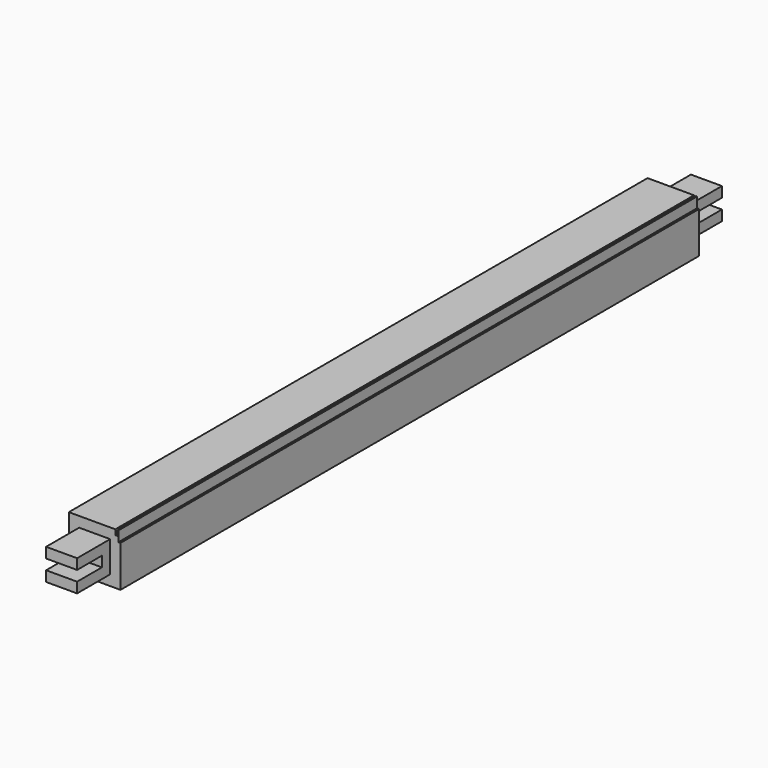
from build123d import *

# Parameters (mm, degrees)
F0_W      = 50
F0_H      = 50
F1_DEPTH  = 700
F3_W      = 30
F3_H      = 30
F4_DEPTH  = 40
F5_W      = 30
F5_H      = 10
F6_DEPTH  = 30
F7_W      = 700
F7_H      = 10
F8_DEPTH  = 2
F9_W      = 2
F9_H      = 700
F10_DEPTH = 5


# Not quite as in the source:
# - a pattern or mirror of a feature is missing from the dataset's text; its kind, count and spacing are read off the source's solid


with BuildPart() as f1:
    # F0 (on Front) → F1 (new body)
    with BuildSketch(Plane.XZ):
        with Locations((-25, 25)):
            Rectangle(F0_W, F0_H)
    extrude(amount=F1_DEPTH)

    # F3 (on face) → F4 (join)
    with BuildSketch(Plane.XZ.offset(700)):
        with Locations((-25, 25)):
            Rectangle(F3_W, F3_H)
    f4 = extrude(amount=F4_DEPTH)

    # F4_copies: F4 across plane
    add(f4.mirror(Plane.ZX.offset(-350)))

    # F5 (on face) → F6 (cut)
    with BuildSketch(Plane.XZ.offset(740)):
        with Locations((-25, 25)):
            Rectangle(F5_W, F5_H)
    f6 = extrude(amount=-F6_DEPTH, mode=Mode.SUBTRACT)

    # F6_copies: F6 across plane
    add(f6.mirror(Plane.ZX.offset(-350)), mode=Mode.SUBTRACT)

    # F7 (on face) → F8 (cut)
    with BuildSketch(Plane.YZ):
        with Locations((-350, 45)):
            Rectangle(F7_W, F7_H)
    extrude(amount=-F8_DEPTH, mode=Mode.SUBTRACT)

    # F9 (on face) → F10 (cut)
    with BuildSketch(Plane.XY.offset(50)):
        with Locations((-4, -350)):
            Rectangle(F9_W, F9_H)
    extrude(amount=-F10_DEPTH, mode=Mode.SUBTRACT)


solid = f1.part
